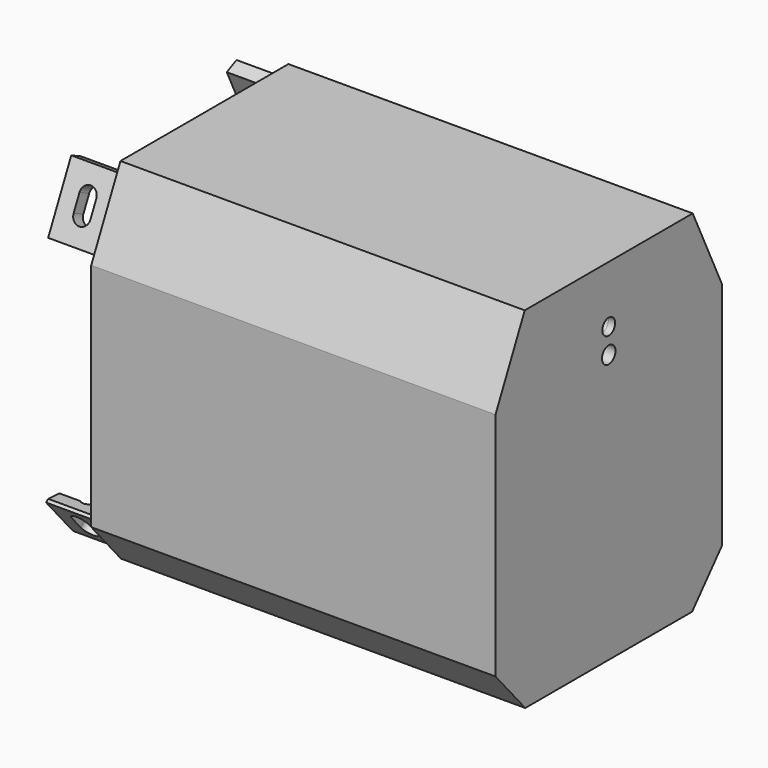
from build123d import *

# Parameters (mm, degrees)
F1_DEPTH       = 152.4
F3_DEPTH       = 2.54
F4_R           = 32.385
F5_DEPTH       = 50.8
F6_R           = 3.175
F6_R_2         = 3.0099
F7_DEPTH       = 7.62
F8_R           = 4.445
F8_R_2         = 3.175
F9_DEPTH       = 127
F10_DEPTH      = 25.4
F11_R          = 1.5875
F12_DEPTH      = 6.35
F14_DEPTH      = 19.05
F14_DEPTH_BACK = 25.4
F16_DEPTH      = 25.4
F18_DEPTH      = 25.4
F19_T1_DEPTH   = 64.0462243683


# Not quite as in the source:
# - a fillet or chamfer that OpenCascade refuses, or shapes differently, is made with other operations: its cross-section is extruded or revolved along the edge and cut away or added
# - a pattern or mirror of a feature is missing from the dataset's text; its kind, count and spacing are read off the source's solid


with BuildPart() as f1:
    # F0 (on Right) → F1 (new body)
    with BuildSketch(Plane.YZ):
        Polygon((53.34, 40.005920294), (39.5708099851, 69.016998145), (-39.5708099851, 69.016998145), (-53.34, 40.005920294), (-53.34, -46.8922357465), (-39.3094271421, -63.063001855), (39.3094271421, -63.063001855), (53.34, -46.8922357465), align=None)
        Polygon((-50.8, -45.9439186117), (-50.8, 39.4337424117), (-37.9647744794, 66.476998145), (37.9647744794, 66.476998145), (50.8, 39.4337424117), (50.8, -45.9439186117), (38.1504515326, -60.523001855), (-38.1504515326, -60.523001855), align=None, mode=Mode.SUBTRACT)
    extrude(amount=F1_DEPTH)

    # F2 (on face) → F3 (join)
    with BuildSketch(Plane.YZ.offset(152.4)):
        Polygon((39.5708099851, 69.016998145), (-39.5708099851, 69.016998145), (-53.34, 40.005920294), (-53.34, -46.8922357465), (-39.3094271421, -63.063001855), (39.3094271421, -63.063001855), (53.34, -46.8922357465), (53.34, 40.005920294), align=None)
    extrude(amount=-F3_DEPTH)

    # F4 (on face) → F5 (join)
    with BuildSketch(Plane(origin=(149.86, 0, 0), x_dir=(0, -1, 0), z_dir=(-1, 0, 0))):
        with BuildLine():
            Line((5.973700434, -60.523001855), (5.973700434, -59.9885985906))
            ThreePointArc((5.973700434, -59.9885985906), (0, 6.786998145), (-5.973700434, -59.9885985906))
            Line((-5.973700434, -59.9885985906), (-5.973700434, -60.523001855))
            Line((-5.973700434, -60.523001855), (5.973700434, -60.523001855))
        make_face()
        with Locations((0, -26.868001855)):
            Circle(F4_R, mode=Mode.SUBTRACT)
    extrude(amount=F5_DEPTH)

    # F6 (on face) → F7 (join)
    with BuildSketch(Plane(origin=(149.86, 0, 0), x_dir=(0, -1, 0), z_dir=(-1, 0, 0))):
        with BuildLine():
            ThreePointArc((3.6918639322, 35.7091109445), (4.2525498338, 36.8908525816), (4.445, 38.1846241653))
            ThreePointArc((4.445, 38.1846241653), (-1.2937715837, 42.4371739991), (-3.6918639322, 35.7091109445))
            ThreePointArc((-3.6918639322, 35.7091109445), (0, 33.7396241653), (3.6918639322, 35.7091109445))
        make_face()
        with Locations((0, 38.1846241653)):
            Circle(F6_R, mode=Mode.SUBTRACT)
        with BuildLine():
            ThreePointArc((-3.6918639322, 35.7091109445), (-1.2937715837, 42.4371739991), (4.445, 38.1846241653))
            ThreePointArc((4.445, 38.1846241653), (4.2525498338, 36.8908525816), (3.6918639322, 35.7091109445))
            ThreePointArc((3.6918639322, 35.7091109445), (4.9935206322, 38.4525755386), (5.4403020609, 41.4561225248))
            Line((5.4403020609, 41.4561225248), (5.4403020609, 49.0812241653))
            ThreePointArc((5.4403020609, 49.0812241653), (4.6963532851, 50.8772753895), (2.9003020609, 51.6212241653))
            Line((2.9003020609, 51.6212241653), (-2.9003020609, 51.6212241653))
            ThreePointArc((-2.9003020609, 51.6212241653), (-4.6963532851, 50.8772753895), (-5.4403020609, 49.0812241653))
            Line((-5.4403020609, 49.0812241653), (-5.4403020609, 41.4561225248))
            ThreePointArc((-5.4403020609, 41.4561225248), (-4.9935206322, 38.4525755386), (-3.6918639322, 35.7091109445))
        make_face()
        with Locations((0, 47.5292321023)):
            Circle(F6_R_2, mode=Mode.SUBTRACT)
    extrude(amount=F7_DEPTH)

    # F8 (on face) → F9 (join)
    with BuildSketch(Plane(origin=(142.24, 0, 0), x_dir=(0, -1, 0), z_dir=(-1, 0, 0))):
        with Locations((0, 38.1846241653)):
            Circle(F8_R)
        with Locations((0, 38.1846241653)):
            Circle(F8_R_2, mode=Mode.SUBTRACT)
    extrude(amount=F9_DEPTH)

    # F10 (cut): faces of the model
    f10_faces = [f1.faces().sort_by_distance(p)[0] for p in [
        (149.86, 0, 47.5292321023),
        (149.86, 0, 38.1846241653),
    ]]
    extrude(f10_faces, amount=-F10_DEPTH, mode=Mode.SUBTRACT)

    # F11 (on face) → F12 (join)
    with BuildSketch(Plane(origin=(0, -50.8, 0), x_dir=(-1, 0, 0), z_dir=(0, 1, 0))):
        with Locations((-52.7279826642, 34.2288921253)):
            Circle(F11_R)
        with Locations((-18.0823826642, 34.2288921253)):
            Circle(F11_R)
        with Locations((-52.7279826642, 6.2126921253)):
            Circle(F11_R)
        with Locations((-18.0823826642, 6.2126921253)):
            Circle(F11_R)
    extrude(amount=F12_DEPTH)

    # F13 (on face) → F14 (join, two sides)
    with BuildSketch(Plane(origin=(0, 0, 0), x_dir=(0, -1, 0), z_dir=(-1, 0, 0))) as f14_sk:
        Polygon((-34.3476103183, 62.2505115972), (-38.9369386243, 64.4286910434), (-49.8278358551, 41.4820495133), (-45.2385075491, 39.3038700672), align=None)
        Polygon((-46.9629683502, -42.6147162871), (-50.8, -45.9439186117), (-38.1504515326, -60.523001855), (-34.3134198828, -57.1937995303), align=None)
        Polygon((45.2385075491, 39.3038700672), (49.8278358551, 41.4820495133), (38.9369386243, 64.4286910434), (34.3476103183, 62.2505115972), align=None)
        Polygon((50.8, -45.9439186117), (46.9629683502, -42.6147162871), (34.3134198828, -57.1937995303), (38.1504515326, -60.523001855), align=None)
    extrude(amount=F14_DEPTH)
    extrude(f14_sk.sketch, amount=-F14_DEPTH_BACK)

    # F15 (on face) → F16 (cut)
    with BuildSketch(Plane(origin=(0, -56.7355756559, 26.927745526), x_dir=(1, 0, 0), z_dir=(0, -0.9034110839, 0.4287754815))):
        with BuildLine():
            Line((-6.35, 25.6353889994), (-6.35, 31.9853889994))
            ThreePointArc((-6.35, 31.9853889994), (-9.525, 35.1603889994), (-12.7, 31.9853889994))
            Line((-12.7, 31.9853889994), (-12.7, 25.6353889994))
            ThreePointArc((-12.7, 25.6353889994), (-9.525, 22.4603889994), (-6.35, 25.6353889994))
        make_face()
    f16 = extrude(amount=-F16_DEPTH, mode=Mode.SUBTRACT)

    # F16_copies: F16 across plane
    add(f16.mirror(Plane.ZX), mode=Mode.SUBTRACT)

    # F17 (on face) → F18 (cut)
    with BuildSketch(Plane(origin=(0, -51.7243071989, -44.878619591), x_dir=(1, 0, 0), z_dir=(0, -0.7553211909, -0.6553547883))):
        with BuildLine():
            Line((-6.35, -14.2363084116), (-6.35, -7.8863084116))
            ThreePointArc((-6.35, -7.8863084116), (-9.525, -4.7113084116), (-12.7, -7.8863084116))
            Line((-12.7, -7.8863084116), (-12.7, -14.2363084116))
            ThreePointArc((-12.7, -14.2363084116), (-9.525, -17.4113084116), (-6.35, -14.2363084116))
        make_face()
    f18 = extrude(amount=-F18_DEPTH, mode=Mode.SUBTRACT)

    # F18_copies: F18 across plane
    add(f18.mirror(Plane.ZX), mode=Mode.SUBTRACT)

    # F19: chamfer of 3.81 on 6 edges, made by hand

    # F19_s2 → F19_t1 (cut)
    with BuildSketch(Plane.YZ.offset(-28.8481121842)):
        Polygon((-48.6805037786, 40.9375046518), (-43.6048729645, 42.7458662967), (-45.2385075491, 39.3038700672), align=None)
        Polygon((48.6805037786, 40.9375046518), (43.6048729645, 42.7458662967), (45.2385075491, 39.3038700672), align=None)
        Polygon((49.8407420876, -45.1116180306), (44.4660666067, -45.4924900244), (46.9629683502, -42.6147162871), align=None)
        Polygon((37.1911936201, -59.6907012738), (36.8103216263, -54.316025793), (34.3134198828, -57.1937995303), align=None)
        Polygon((-49.8407420876, -45.1116180306), (-44.4660666067, -45.4924900244), (-46.9629683502, -42.6147162871), align=None)
        Polygon((-37.1911936201, -59.6907012738), (-36.8103216263, -54.316025793), (-34.3134198828, -57.1937995303), align=None)
    extrude(amount=F19_T1_DEPTH, mode=Mode.SUBTRACT)


solid = f1.part
